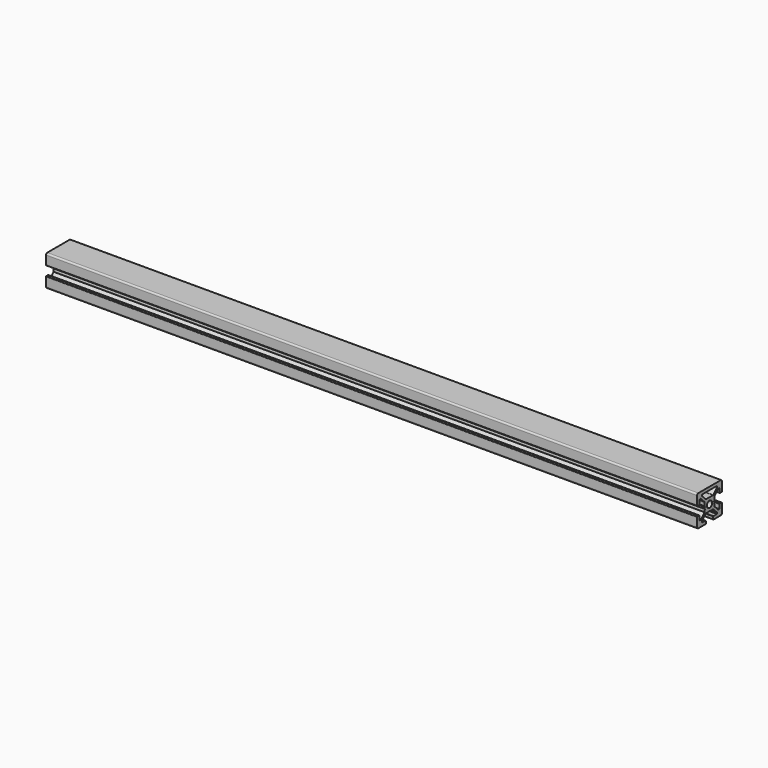
from build123d import *

# Parameters (mm, degrees)
F1_DEPTH = 210


# Not quite as in the source:
# - ends of sketch curves that miss each other by under 0.0002 mm in the source are joined


with BuildPart() as f1:
    # F0 (on Right) → F1 (new body, symmetric)
    with BuildSketch(Plane.YZ):
        with BuildLine():
            Line((9.043565, 10.073321), (0.043565, 10.073321))
            Line((0.043565, 10.073321), (-8.956435, 10.073321))
            ThreePointArc((-8.956435, 10.073321), (-9.6635417812, 9.7804277812), (-9.956435, 9.073321))
            Line((-9.956435, 9.073321), (-9.956435, 3.373321))
            ThreePointArc((-9.956435, 3.373321), (-9.8685670344, 3.1611889656), (-9.656435, 3.073321))
            Line((-9.656435, 3.073321), (-8.256435, 3.073321))
            ThreePointArc((-8.256435, 3.073321), (-8.0443029656, 3.1611889656), (-7.956435, 3.373321))
            Line((-7.956435, 3.373321), (-7.956435, 6.073321))
            Line((-7.956435, 6.073321), (-7.017095, 6.073321))
            Line((-7.017095, 6.073321), (-3.956435, 3.012661))
            Line((-3.956435, 3.012661), (-3.956435, 0.726911))
            ThreePointArc((-3.956435, 0.726911), (-3.9393979324, 0.5975015494), (-3.8894477764, 0.4769111291))
            Line((-3.8894477764, 0.4769111291), (-3.656435, 0.073321))
            Line((-3.656435, 0.073321), (-3.889448, -0.330269))
            ThreePointArc((-3.889448, -0.330269), (-3.956435, -0.580269), (-3.8894477764, -0.8302688709))
            Line((-3.8894477764, -0.8302688709), (-3.707412, -1.145565))
            Line((-3.707412, -1.145565), (-3.956435, -2.426679))
            Line((-3.956435, -2.426679), (-3.956435, -2.866019))
            Line((-3.956435, -2.866019), (-7.017095, -5.926679))
            Line((-7.017095, -5.926679), (-7.956435, -5.926679))
            Line((-7.956435, -5.926679), (-7.956435, -3.226679))
            ThreePointArc((-7.956435, -3.226679), (-8.0443029656, -3.0145469656), (-8.256435, -2.926679))
            Line((-8.256435, -2.926679), (-9.656435, -2.926679))
            ThreePointArc((-9.656435, -2.926679), (-9.8685670344, -3.0145469656), (-9.956435, -3.226679))
            Line((-9.956435, -3.226679), (-9.956435, -8.926679))
            ThreePointArc((-9.956435, -8.926679), (-9.6635417812, -9.6337857812), (-8.956435, -9.926679))
            Line((-8.956435, -9.926679), (-3.256435, -9.926679))
            ThreePointArc((-3.256435, -9.926679), (-3.0443029656, -9.8388110344), (-2.956435, -9.626679))
            Line((-2.956435, -9.626679), (-2.956435, -8.226679))
            ThreePointArc((-2.956435, -8.226679), (-3.0443029656, -8.0145469656), (-3.256435, -7.926679))
            Line((-3.256435, -7.926679), (-5.956435, -7.926679))
            Line((-5.956435, -7.926679), (-5.956435, -6.987339))
            Line((-5.956435, -6.987339), (-2.895775, -3.926679))
            Line((-2.895775, -3.926679), (-0.610025, -3.926679))
            ThreePointArc((-0.610025, -3.926679), (-0.4806155494, -3.9096419324), (-0.3600251291, -3.8596917764))
            Line((-0.3600251291, -3.8596917764), (-0.0645959325, -3.6891257984))
            Line((-0.0645959325, -3.6891257984), (0.2217128734, -3.8544264098))
            ThreePointArc((0.2217128734, -3.8544264098), (0.3921793907, -3.9150473077), (0.5730594828, -3.9110345539))
            ThreePointArc((0.5730594828, -3.9110345539), (0.6346161199, -3.9227524708), (0.697155, -3.926679))
            Line((0.697155, -3.926679), (2.982905, -3.926679))
            Line((2.982905, -3.926679), (6.043565, -6.987339))
            Line((6.043565, -6.987339), (6.043565, -7.926679))
            Line((6.043565, -7.926679), (3.343565, -7.926679))
            ThreePointArc((3.343565, -7.926679), (3.1314329656, -8.0145469656), (3.043565, -8.226679))
            Line((3.043565, -8.226679), (3.043565, -9.626679))
            ThreePointArc((3.043565, -9.626679), (3.1314329656, -9.8388110344), (3.343565, -9.926679))
            Line((3.343565, -9.926679), (9.043565, -9.926679))
            ThreePointArc((9.043565, -9.926679), (9.7506717812, -9.6337857812), (10.043565, -8.926679))
            Line((10.043565, -8.926679), (10.043565, -3.226679))
            ThreePointArc((10.043565, -3.226679), (9.9556970344, -3.0145469656), (9.743565, -2.926679))
            Line((9.743565, -2.926679), (8.343565, -2.926679))
            ThreePointArc((8.343565, -2.926679), (8.1314329656, -3.0145469656), (8.043565, -3.226679))
            Line((8.043565, -3.226679), (8.043565, -5.926679))
            Line((8.043565, -5.926679), (7.104225, -5.926679))
            Line((7.104225, -5.926679), (4.043565, -2.866019))
            Line((4.043565, -2.866019), (4.043565, -2.426679))
            Line((4.043565, -2.426679), (3.794542, -1.145565))
            Line((3.794542, -1.145565), (3.976578, -0.830269))
            ThreePointArc((3.976578, -0.830269), (4.043565, -0.580269), (3.9765777764, -0.3302691291))
            Line((3.9765777764, -0.3302691291), (3.743565, 0.073321))
            Line((3.743565, 0.073321), (3.976578, 0.476911))
            ThreePointArc((3.976578, 0.476911), (4.0265279324, 0.5975015494), (4.043565, 0.726911))
            Line((4.043565, 0.726911), (4.043565, 3.012661))
            Line((4.043565, 3.012661), (7.104225, 6.073321))
            Line((7.104225, 6.073321), (8.043565, 6.073321))
            Line((8.043565, 6.073321), (8.043565, 3.373321))
            ThreePointArc((8.043565, 3.373321), (8.1314329656, 3.1611889656), (8.343565, 3.073321))
            Line((8.343565, 3.073321), (9.743565, 3.073321))
            ThreePointArc((9.743565, 3.073321), (9.9556970344, 3.1611889656), (10.043565, 3.373321))
            Line((10.043565, 3.373321), (10.043565, 9.073321))
            ThreePointArc((10.043565, 9.073321), (9.7506717812, 9.7804277812), (9.043565, 10.073321))
        make_face()
        with BuildLine():
            ThreePointArc((0.043565, 2.173321), (2.143565, 0.073321), (0.043565, -2.026679))
            ThreePointArc((0.043565, -2.026679), (-2.056435, 0.073321), (0.043565, 2.173321))
        make_face(mode=Mode.SUBTRACT)
        with BuildLine():
            Line((2.775798, 4.073321), (0.043565, 4.073321))
            Line((0.043565, 4.073321), (-2.688668, 4.073321))
            ThreePointArc((-2.688668, 4.073321), (-2.8800097162, 4.1113812337), (-3.0422213906, 4.2197676094))
            Line((-3.0422213906, 4.2197676094), (-5.809988, 6.987535))
            ThreePointArc((-5.809988, 6.987535), (-5.9183747663, 7.1497462838), (-5.956435, 7.341088))
            Line((-5.956435, 7.341088), (-5.956435, 7.573321))
            ThreePointArc((-5.956435, 7.573321), (-5.8099883906, 7.9268743906), (-5.456435, 8.073321))
            Line((-5.456435, 8.073321), (0.043565, 8.073321))
            Line((0.043565, 8.073321), (5.543565, 8.073321))
            ThreePointArc((5.543565, 8.073321), (5.8971183906, 7.9268743906), (6.043565, 7.573321))
            Line((6.043565, 7.573321), (6.043565, 7.341088))
            ThreePointArc((6.043565, 7.341088), (6.0055047663, 7.1497462838), (5.8971183906, 6.9875346094))
            Line((5.8971183906, 6.9875346094), (3.129351, 4.219768))
            ThreePointArc((3.129351, 4.219768), (2.9671397162, 4.1113812337), (2.775798, 4.073321))
        make_face(mode=Mode.SUBTRACT)
    extrude(amount=F1_DEPTH, both=True)


solid = f1.part
